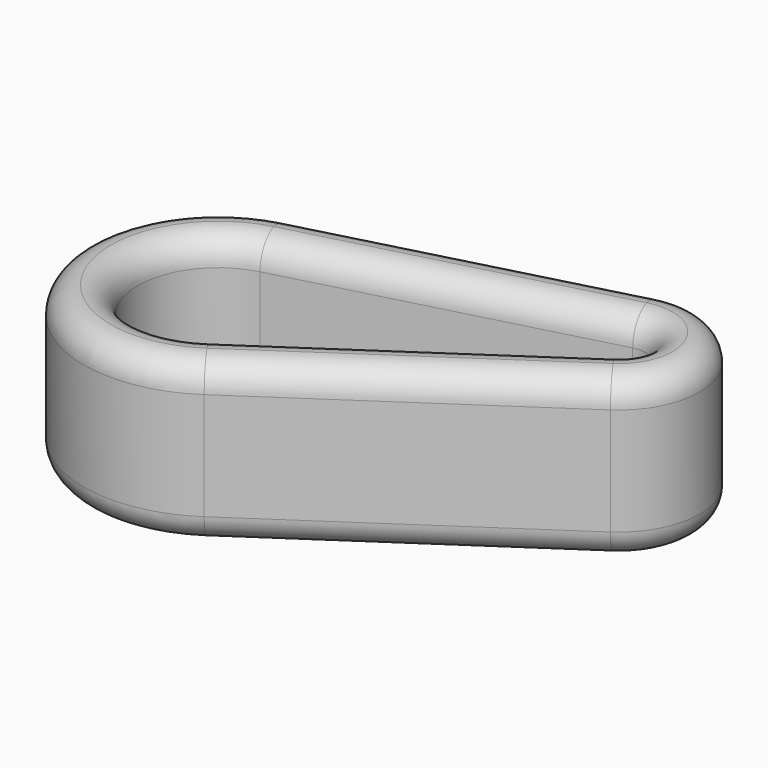
from build123d import *

# Parameters (mm, degrees)
F1_DEPTH = 29.972
F2_R     = 4.99999


# Not quite as in the source:
# - a fillet or chamfer is up to 0.001 mm smaller than in the source, because OpenCascade refuses the exact size


with BuildPart() as f1:
    # F0 (on Top) → F1 (new body)
    with BuildSketch(Plane.XY):
        with BuildLine():
            Line((50.8110900275, 39.270053991), (-6.3821109307, 24.1650305406))
            ThreePointArc((-6.3821109307, 24.1650305406), (-22.7618789315, -10.3236092753), (13.9758283727, -20.7209136444))
            Line((13.9758283727, -20.7209136444), (63.0175780244, 12.3567337988))
            ThreePointArc((63.0175780244, 12.3567337988), (68.2856367944, 30.9708278258), (50.8110900275, 39.270053991))
        make_face()
        with BuildLine():
            ThreePointArc((8.3840655323, -12.4304258217), (-13.6547959456, -6.1931081569), (-3.8286128629, 14.4965431916))
            Line((-3.8286128629, 14.4965431916), (53.3645880953, 29.601566642))
            ThreePointArc((53.3645880953, 29.601566642), (59.1785538086, 26.8403267074), (57.4258151841, 20.6472216214))
            Line((57.4258151841, 20.6472216214), (8.3840655323, -12.4304258217))
        make_face(mode=Mode.SUBTRACT)
    extrude(amount=F1_DEPTH)

    # F2 (radius 5 in the source; OpenCascade refuses exactly that, so slightly less here)
    f2_edges = [f1.edges().sort_by_distance(p)[0] for p in [
        (22.21449, 31.717542, 29.972),
        (-22.761879, -10.323609, 29.972),
        (38.496703, -4.18209, 29.972),
        (68.285637, 30.970828, 29.972),
        (59.178554, 26.840327, 29.972),
        (32.90494, 4.108398, 29.972),
        (-13.654796, -6.193108, 29.972),
        (24.767988, 22.049055, 29.972),
        (22.21449, 31.717542, 0),
        (-22.761879, -10.323609, 0),
        (38.496703, -4.18209, 0),
        (68.285637, 30.970828, 0),
        (59.178554, 26.840327, 0),
        (32.90494, 4.108398, 0),
        (-13.654796, -6.193108, 0),
        (24.767988, 22.049055, 0),
    ]]
    fillet(f2_edges, radius=F2_R)


solid = f1.part
